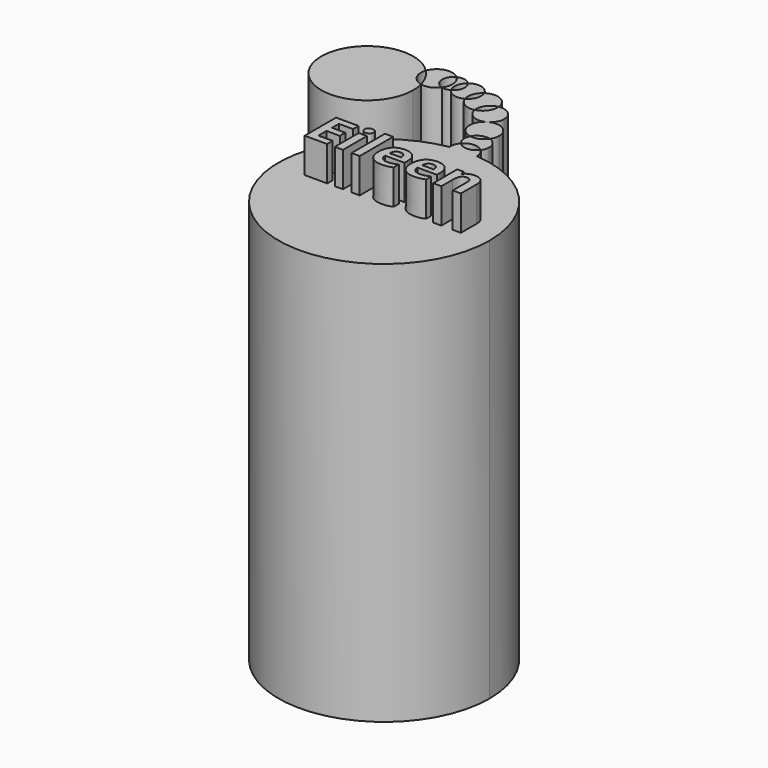
from build123d import *

# Parameters (mm, degrees)
F1_DEPTH     = 12.7
F2_TEXT_SIZE = 1.7310078773
F3_DEPTH     = 1.0922


# Not quite as in the source:
# - Text() gives the source's letters only with a copy of the font that has no kerning and outlines rounded to 1/6400 em; it was checked with that copy


with BuildPart() as f1:
    # F0 (on Top) → F1 (new body)
    with BuildSketch(Plane.XY):
        with BuildLine():
            ThreePointArc((0.8550593898, 13.7235949023), (-0.7241423285, 7.9037908659), (4.7438161887, 10.446511209))
            ThreePointArc((4.7438161887, 10.446511209), (3.8635159685, 12.7002640163), (1.6887111288, 13.7607139695))
            ThreePointArc((1.6887111288, 13.7607139695), (1.2893125455, 13.3507575468), (0.8550593898, 13.7235949023))
        make_face()
        with BuildLine():
            ThreePointArc((0.8550593898, 13.7235949023), (1.2893125455, 13.3507575468), (1.6887111288, 13.7607139695))
            ThreePointArc((1.6887111288, 13.7607139695), (1.2707162309, 13.7684094742), (0.8550593898, 13.7235949023))
        make_face()
        with BuildLine():
            ThreePointArc((0.8550593898, 13.7235949023), (1.2707162309, 13.7684094742), (1.6887111288, 13.7607139695))
            ThreePointArc((1.6887111288, 13.7607139695), (1.6887642532, 13.7645615589), (1.6887819619, 13.7684094742))
            ThreePointArc((1.6887819619, 13.7684094742), (1.6544554614, 13.9343105243), (1.5571129139, 14.0729679997))
            ThreePointArc((1.5571129139, 14.0729679997), (1.2643499892, 13.9209823841), (0.9599432943, 14.0480505608))
            ThreePointArc((0.9599432943, 14.0480505608), (0.8729186391, 13.8970019753), (0.8550593898, 13.7235949023))
        make_face()
    extrude(amount=F1_DEPTH)

    # F2 (on face) → F3 (join)
    with BuildSketch(Plane.XY.offset(12.7)):
        with Locations((-1.1444879929, 10.3274099529)):
            Text('Eileen', F2_TEXT_SIZE, font='Open Sans', font_style=FontStyle.BOLD, text_align=(TextAlign.LEFT, TextAlign.BOTTOM))
    extrude(amount=F3_DEPTH)


with BuildPart() as f1b:
    # F0 (on Top) → F1, piece 2 (new body)
    with BuildSketch(Plane.XY):
        with BuildLine():
            ThreePointArc((0.899897807, 14.4849451595), (0.8621514876, 14.2571838827), (0.9599432943, 14.0480505608))
            ThreePointArc((0.9599432943, 14.0480505608), (1.2532872285, 14.186111743), (1.5571129139, 14.0729679997))
            ThreePointArc((1.5571129139, 14.0729679997), (1.6169985475, 14.1849431558), (1.6376932951, 14.3102286384))
            ThreePointArc((1.6376932951, 14.3102286384), (1.5622352482, 14.5406645794), (1.3650917886, 14.68183503))
            ThreePointArc((1.3650917886, 14.68183503), (1.161615681, 14.5145858461), (0.899897807, 14.4849451595))
        make_face()
    extrude(amount=F1_DEPTH)


with BuildPart() as f1c:
    # F0 (on Top) → F1, piece 3 (new body)
    with BuildSketch(Plane.XY):
        with BuildLine():
            ThreePointArc((0.697112057, 15.3097751115), (0.5298064627, 14.8313001913), (0.899897807, 14.4849451595))
            ThreePointArc((0.899897807, 14.4849451595), (1.0962600722, 14.6690023015), (1.3650917886, 14.68183503))
            ThreePointArc((1.3650917886, 14.68183503), (1.4245221373, 14.8060043811), (1.4449303097, 14.9421421811))
            ThreePointArc((1.4449303097, 14.9421421811), (1.2433372408, 15.3249598092), (0.813625812, 15.3753303352))
            ThreePointArc((0.813625812, 15.3753303352), (0.7578842142, 15.3380822226), (0.697112057, 15.3097751115))
        make_face()
    extrude(amount=F1_DEPTH)


with BuildPart() as f1d:
    # F0 (on Top) → F1, piece 4 (new body)
    with BuildSketch(Plane.XY):
        with BuildLine():
            ThreePointArc((0.1103541708, 15.6513124221), (0.322664178, 15.3412680976), (0.697112057, 15.3097751115))
            ThreePointArc((0.697112057, 15.3097751115), (0.752996967, 15.3467685101), (0.813625812, 15.3753303352))
            ThreePointArc((0.813625812, 15.3753303352), (0.9370589181, 15.5283304503), (0.9811632967, 15.7199017704))
            ThreePointArc((0.9811632967, 15.7199017704), (0.8253499564, 16.0549355817), (0.4687406883, 16.1516582866))
            ThreePointArc((0.4687406883, 16.1516582866), (0.4702013003, 16.1302921462), (0.4706885072, 16.1088816822))
            ThreePointArc((0.4706885072, 16.1088816822), (0.369790556, 15.8176727959), (0.1103541708, 15.6513124221))
        make_face()
    extrude(amount=F1_DEPTH)


with BuildPart() as f1e:
    # F0 (on Top) → F1, piece 5 (new body)
    with BuildSketch(Plane.XY):
        with BuildLine():
            ThreePointArc((-0.4475574125, 15.9631420743), (-0.2296430699, 15.698014634), (0.1103541708, 15.6513124221))
            ThreePointArc((0.1103541708, 15.6513124221), (0.1868920194, 15.9750151215), (0.4687406883, 16.1516582866))
            ThreePointArc((0.4687406883, 16.1516582866), (0.1994690795, 16.5352146003), (-0.2675384239, 16.4961423986))
            ThreePointArc((-0.2675384239, 16.4961423986), (-0.2409128728, 16.4137846445), (-0.2319077231, 16.3276996464))
            ThreePointArc((-0.2319077231, 16.3276996464), (-0.2898565935, 16.1159173218), (-0.4475574125, 15.9631420743))
        make_face()
    extrude(amount=F1_DEPTH)


with BuildPart() as f1f:
    # F0 (on Top) → F1, piece 6 (new body)
    with BuildSketch(Plane.XY):
        with BuildLine():
            ThreePointArc((-1.0043900725, 16.1133917612), (-0.7562412199, 15.9260941718), (-0.4475574125, 15.9631420743))
            ThreePointArc((-0.4475574125, 15.9631420743), (-0.4459404111, 16.2594964907), (-0.2675384239, 16.4961423986))
            ThreePointArc((-0.2675384239, 16.4961423986), (-0.5484571157, 16.7316126526), (-0.9065770483, 16.6534355086))
            ThreePointArc((-0.9065770483, 16.6534355086), (-0.843376687, 16.5459433106), (-0.821399681, 16.4232002068))
            ThreePointArc((-0.821399681, 16.4232002068), (-0.8705636395, 16.2432927609), (-1.0043900725, 16.1133917612))
        make_face()
    extrude(amount=F1_DEPTH)


with BuildPart() as f1g:
    # F0 (on Top) → F1, piece 7 (new body)
    with BuildSketch(Plane.XY):
        with BuildLine():
            ThreePointArc((-1.2697047373, 16.0823175483), (-1.1340015635, 16.0718489636), (-1.0043900725, 16.1133917612))
            ThreePointArc((-1.0043900725, 16.1133917612), (-1.0571855349, 16.4018339532), (-0.9065770483, 16.6534355086))
            ThreePointArc((-0.9065770483, 16.6534355086), (-1.1043782299, 16.7698009781), (-1.3319651272, 16.7402978576))
            ThreePointArc((-1.3319651272, 16.7402978576), (-1.2144393145, 16.5750220389), (-1.1729485019, 16.3765102625))
            ThreePointArc((-1.1729485019, 16.3765102625), (-1.1977585216, 16.2216626582), (-1.2697047373, 16.0823175483))
        make_face()
    extrude(amount=F1_DEPTH)


with BuildPart() as f1h:
    # F0 (on Top) → F1, piece 8 (new body)
    with BuildSketch(Plane.XY):
        with BuildLine():
            ThreePointArc((-1.7754142255, 15.8925282747), (-1.4944337617, 15.9124795649), (-1.2697047373, 16.0823175483))
            ThreePointArc((-1.2697047373, 16.0823175483), (-1.5273323173, 16.389875731), (-1.3319651272, 16.7402978576))
            ThreePointArc((-1.3319651272, 16.7402978576), (-1.7907848465, 16.8568415345), (-2.1381233272, 16.5351989638))
            ThreePointArc((-2.1381233272, 16.5351989638), (-1.9151066757, 16.237376786), (-1.7754142255, 15.8925282747))
        make_face()
    extrude(amount=F1_DEPTH)


with BuildPart() as f1i:
    # F0 (on Top) → F1, piece 9 (new body)
    with BuildSketch(Plane.XY):
        with BuildLine():
            ThreePointArc((-1.7282808945, 15.5262360349), (-1.7401126039, 15.710892172), (-1.7754142255, 15.8925282747))
            ThreePointArc((-1.7754142255, 15.8925282747), (-2.100215888, 16.1329052468), (-2.1381233272, 16.5351989638))
            ThreePointArc((-2.1381233272, 16.5351989638), (-4.515649168, 14.9817231766), (-1.7282808945, 15.5262360349))
        make_face()
    extrude(amount=F1_DEPTH)


solid = Compound([f1.part, f1b.part, f1c.part, f1d.part, f1e.part, f1f.part, f1g.part, f1h.part, f1i.part])
